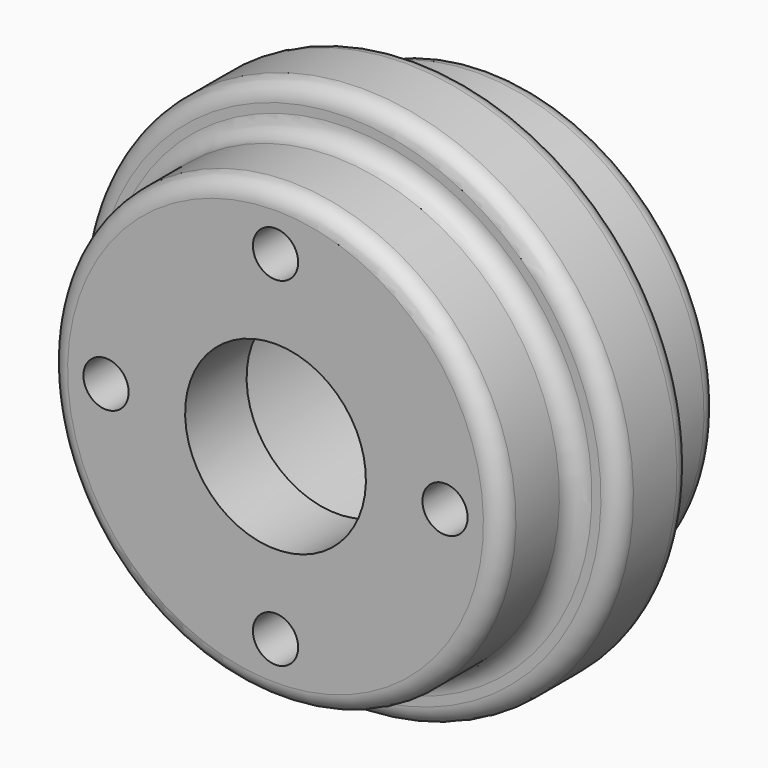
from build123d import *

# Parameters (mm, degrees)
F0_W             = 21.59
F0_H             = 12.7
F2_R             = 5.08
F3_R             = 6.35
F4_DEPTH         = 25.4
F4_COPIES_COUNT  = 4
F4_COPIES2_COUNT = 2
F4_COPIES2_PITCH = 84.361847
F4_COPIES3_COUNT = 2
F4_COPIES3_PITCH = 84.361847
F4_COPIES4_COUNT = 2
F4_COPIES4_PITCH = 107.95


# Not quite as in the source:
# - a pattern or mirror of a feature is missing from the dataset's text; its kind, count and spacing are read off the source's solid


with BuildPart() as f1:
    # F0 (on Right) → F1 (revolve)
    with BuildSketch(Plane.YZ):
        Polygon((-38.1, 63.5), (-38.1, 38.1), (-16.51, 38.1), (38.1, 38.1), (38.1, 63.5), (12.7, 63.5), (12.7, 76.2), (-12.7, 76.2), (-12.7, 63.5), align=None)
        with Locations((-27.305, 31.75)):
            Rectangle(F0_W, F0_H)
    revolve(axis=Axis((0, 4.9274371037, 0), (0, 1, 0)))

    # F2
    f2_edges = [f1.edges().sort_by_distance(p)[0] for p in [
        (0, -12.7, -63.5),
        (0, -12.7, -76.2),
        (0, 12.7, -76.2),
        (0, 38.1, -63.5),
        (0, -38.1, -63.5),
    ]]
    fillet(f2_edges, radius=F2_R)

    # F3 (on face) → F4 (cut)
    with BuildSketch(Plane(origin=(0, 38.1, 0), x_dir=(-1, 0, 0), z_dir=(0, 1, 0))):
        with Locations((0, 47.625)):
            Circle(F3_R)
    f4 = extrude(amount=-F4_DEPTH, mode=Mode.SUBTRACT)

    # F4_copies: F4 ×4 about axis
    f4_copies_axis = Axis((0, 0, 0), (0, 1, 0))
    for i in range(1, F4_COPIES_COUNT):
        add(f4.rotate(f4_copies_axis, i * 360 / F4_COPIES_COUNT), mode=Mode.SUBTRACT)

    # F4_copies1: F4 across plane
    add(f4.mirror(Plane(origin=(0, 0, 0), x_dir=(0, 0, -1), z_dir=(0, -1, 0))), mode=Mode.SUBTRACT)

    # F4_copies2: F4 ×2
    with Locations(*[Vector(0.5645324471, -0.6021679436, -0.5645324471) * (i * F4_COPIES2_PITCH) for i in range(1, F4_COPIES2_COUNT)]):
        add(f4, mode=Mode.SUBTRACT)

    # F4_copies3: F4 ×2
    with Locations(*[Vector(-0.5645324471, -0.6021679436, -0.5645324471) * (i * F4_COPIES3_PITCH) for i in range(1, F4_COPIES3_COUNT)]):
        add(f4, mode=Mode.SUBTRACT)

    # F4_copies4: F4 ×2
    with Locations(*[Vector(0, -0.4705882353, -0.8823529412) * (i * F4_COPIES4_PITCH) for i in range(1, F4_COPIES4_COUNT)]):
        add(f4, mode=Mode.SUBTRACT)


solid = f1.part
